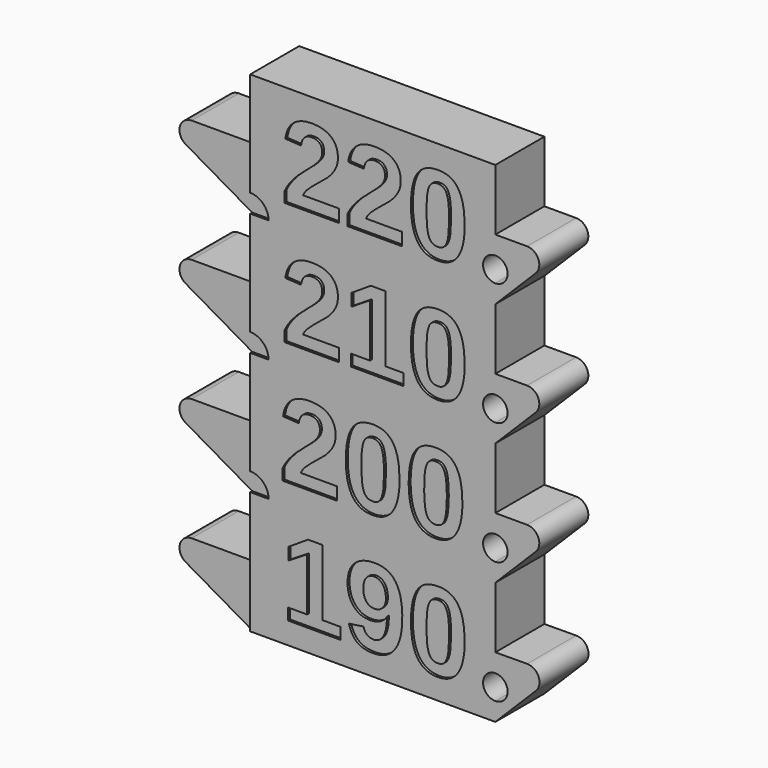
from build123d import *
from build123d import SkipClean  # not in build123d's __all__

# Parameters (mm, degrees)
F1_DEPTH     = 40
F3_DEPTH     = 5
F2_TEXT_SIZE = 9.217474796
F4_DEPTH     = 0.2
F5_R         = 1
F6_DEPTH     = 5.001


# Not quite as in the source:
# - Text() gives the source's letters only with a copy of the font that has no kerning and outlines rounded to 1/6400 em; it was checked with that copy


with BuildPart() as f1:
    # F0 (on Top) → F1 (new body)
    with BuildSketch(Plane.XY):
        Polygon((-7, 2.5), (-10, 2.5), (-10, -2.5), (10, -2.5), (10, 2.5), (7, 2.5), align=None)
    extrude(amount=F1_DEPTH)

    # F2 (on face) → F3 (join)
    with BuildSketch(Plane.XZ.offset(2.5)):
        Polygon((-18.6602540378, 35), (-10, 30), (-10, 31.5), (-10, 35), align=None)
        Polygon((-18.6602540378, 25), (-10, 20), (-10, 21.5), (-10, 25), align=None)
        with BuildLine():
            Line((10, 21.5), (10, 20))
            Line((10, 20), (15, 25))
            Line((15, 25), (10, 25))
            Line((10, 25), (10, 23.5))
            ThreePointArc((10, 23.5), (10.7071067812, 23.2071067812), (11, 22.5))
            ThreePointArc((11, 22.5), (10.7071067812, 21.7928932188), (10, 21.5))
        make_face()
        Polygon((-18.6602540378, 15), (-10, 10), (-10, 11.5), (-10, 15), align=None)
        Polygon((-10, 0), (-10, 5), (-18.6602540378, 5), align=None)
        with BuildLine():
            Line((10, 11.5), (10, 10))
            Line((10, 10), (15, 15))
            Line((15, 15), (10, 15))
            Line((10, 15), (10, 13.5))
            ThreePointArc((10, 13.5), (10.7071067812, 13.2071067812), (11, 12.5))
            ThreePointArc((11, 12.5), (10.7071067812, 11.7928932188), (10, 11.5))
        make_face()
        with BuildLine():
            Line((10, 31.5), (10, 30))
            Line((10, 30), (15, 35))
            Line((15, 35), (10, 35))
            Line((10, 35), (10, 33.5))
            ThreePointArc((10, 33.5), (10.7071067812, 33.2071067812), (11, 32.5))
            ThreePointArc((11, 32.5), (10.7071067812, 31.7928932188), (10, 31.5))
        make_face()
        with BuildLine():
            Line((15.0323364424, 5.0323364424), (10, 5))
            Line((10, 5), (10, 3.5))
            ThreePointArc((10, 3.5), (10.7071067812, 3.2071067812), (11, 2.5))
            ThreePointArc((11, 2.5), (10.7071067812, 1.7928932188), (10, 1.5))
            Line((10, 1.5), (10, 0))
            Line((10, 0), (15.0323364424, 5.0323364424))
        make_face()
    extrude(amount=-F3_DEPTH)

    # F2 (on face) → F4 (cut)
    with BuildSketch(Plane.XZ.offset(2.5)):
        with BuildLine():
            Line((-10, 11.5), (-10, 10))
            Line((-10, 10), (-8.5, 10))
            ThreePointArc((-8.5, 10), (-8.9393398282, 11.0606601718), (-10, 11.5))
        make_face()
        Polygon((-18.6602540378, 15), (-10, 10), (-10, 11.5), (-10, 15), align=None)
        Polygon((-10, 0), (-10, 5), (-18.6602540378, 5), align=None)
        with BuildLine():
            ThreePointArc((11, 32.5), (9.2928932188, 33.2071067812), (10, 31.5))
            ThreePointArc((10, 31.5), (10.7071067812, 31.7928932188), (11, 32.5))
        make_face()
        Polygon((-18.6602540378, 35), (-10, 30), (-10, 31.5), (-10, 35), align=None)
        with BuildLine():
            Line((-10, 31.5), (-10, 30))
            Line((-10, 30), (-8.5, 30))
            ThreePointArc((-8.5, 30), (-8.9393398282, 31.0606601718), (-10, 31.5))
        make_face()
        with BuildLine():
            ThreePointArc((11, 22.5), (9.2928932188, 23.2071067812), (10, 21.5))
            ThreePointArc((10, 21.5), (10.7071067812, 21.7928932188), (11, 22.5))
        make_face()
        Polygon((-18.6602540378, 25), (-10, 20), (-10, 21.5), (-10, 25), align=None)
        with BuildLine():
            Line((-10, 21.5), (-10, 20))
            Line((-10, 20), (-8.5, 20))
            ThreePointArc((-8.5, 20), (-8.9393398282, 21.0606601718), (-10, 21.5))
        make_face()
        with BuildLine():
            ThreePointArc((11, 12.5), (9.2928932188, 13.2071067812), (10, 11.5))
            ThreePointArc((10, 11.5), (10.7071067812, 11.7928932188), (11, 12.5))
        make_face()
        with BuildLine():
            ThreePointArc((10, 1.5), (10.7071067812, 1.7928932188), (11, 2.5))
            ThreePointArc((11, 2.5), (9.2928932188, 3.2071067812), (10, 1.5))
        make_face()
        with Locations((-7.5, 1.78141072)):
            Text('190', F2_TEXT_SIZE, font='Arimo', font_style=FontStyle.BOLD, text_align=(TextAlign.LEFT, TextAlign.BOTTOM))
        with Locations((-7.6868166897, 11.6817090735)):
            Text('200', F2_TEXT_SIZE, font='Arimo', font_style=FontStyle.BOLD, text_align=(TextAlign.LEFT, TextAlign.BOTTOM))
        with Locations((-7.5, 21.6817090735)):
            Text('210', F2_TEXT_SIZE, font='Arimo', font_style=FontStyle.BOLD, text_align=(TextAlign.LEFT, TextAlign.BOTTOM))
        with Locations((-7.5, 31.6817090735)):
            Text('220', F2_TEXT_SIZE, font='Arimo', font_style=FontStyle.BOLD, text_align=(TextAlign.LEFT, TextAlign.BOTTOM))
    with SkipClean():  # cleaning this boolean's faces spoils the solid; the shape is the same uncleaned
        extrude(amount=-F4_DEPTH, mode=Mode.SUBTRACT)

    # F5
    f5_edges = [f1.edges().sort_by_distance(p)[0] for p in [
        (15, 0, 35),
        (15, 0, 25),
        (15, 0, 15),
        (15.032336, 0, 5.032336),
        (-18.660254, 0.1, 5),
        (-18.660254, 0.1, 15),
        (-18.660254, 0.1, 25),
        (-18.660254, 0.1, 35),
    ]]
    fillet(f5_edges, radius=F5_R)

    # F2 (on face) → F6 (cut, through all)
    with BuildSketch(Plane.XZ.offset(2.5)):
        with BuildLine():
            ThreePointArc((10, 13.5), (9, 12.5), (10, 11.5))
            Line((10, 11.5), (10, 13.5))
        make_face()
        with BuildLine():
            Line((10, 1.5), (10, 3.5))
            ThreePointArc((10, 3.5), (9, 2.5), (10, 1.5))
        make_face()
        with BuildLine():
            ThreePointArc((11, 2.5), (10.7071067812, 3.2071067812), (10, 3.5))
            Line((10, 3.5), (10, 1.5))
            ThreePointArc((10, 1.5), (10.7071067812, 1.7928932188), (11, 2.5))
        make_face()
        with BuildLine():
            ThreePointArc((10, 23.5), (9, 22.5), (10, 21.5))
            Line((10, 21.5), (10, 23.5))
        make_face()
        with BuildLine():
            ThreePointArc((10, 33.5), (9, 32.5), (10, 31.5))
            Line((10, 31.5), (10, 33.5))
        make_face()
    extrude(amount=-F6_DEPTH, mode=Mode.SUBTRACT)


solid = f1.part
